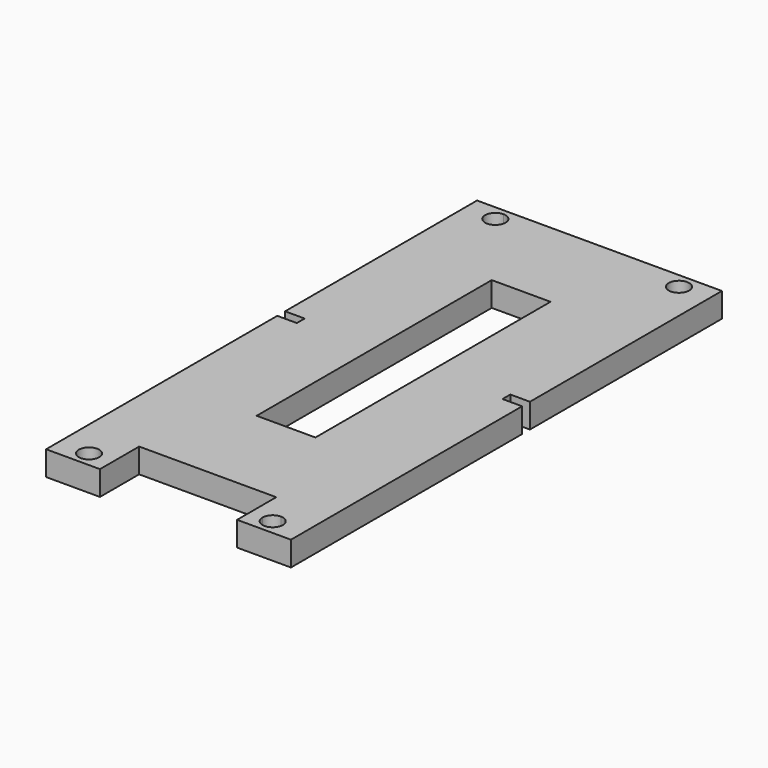
from build123d import *

# Parameters (mm, degrees)
F1_DEPTH  = 3.175
F2_W      = 1.27
F2_H      = 3.175
F3_DEPTH  = 2.54
F4_W      = 1.27
F4_H      = 3.175
F5_DEPTH  = 2.54
F6_W      = 6.985
F6_H      = 3.175
F7_DEPTH  = 6.35
F9_DEPTH  = 25.4
F10_DEPTH = 25.4


# Not quite as in the source:
# - a feature names something its author has since deleted; it is built from what else it names


with BuildPart() as f1:
    # F0 (on Top) → F1 (new body)
    with BuildSketch(Plane.XY):
        Polygon((0, 63.5), (0, 0), (15.875, 0), (15.875, 12.7), (12.065, 12.7), (12.065, 50.8), (15.875, 50.8), (15.875, 63.5), align=None)
        Polygon((15.875, 12.7), (15.875, 0), (31.75, 0), (31.75, 63.5), (15.875, 63.5), (15.875, 50.8), (19.685, 50.8), (19.685, 12.7), align=None)
    extrude(amount=F1_DEPTH)

    # F2 (on face) → F3 (cut)
    with BuildSketch(Plane.YZ.offset(31.75)):
        with Locations((31.75, 1.5875)):
            Rectangle(F2_W, F2_H)
    extrude(amount=-F3_DEPTH, mode=Mode.SUBTRACT)

    # F4 (on face) → F5 (cut)
    with BuildSketch(Plane(origin=(0, 0, 0), x_dir=(0, -1, 0), z_dir=(-1, 0, 0))):
        with Locations((-31.75, 1.5875)):
            Rectangle(F4_W, F4_H)
    extrude(amount=-F5_DEPTH, mode=Mode.SUBTRACT)

    # F6 (on face) → F7 (join)
    with BuildSketch(Plane.XZ):
        with Locations((3.4925, 1.5875)):
            Rectangle(F6_W, F6_H)
        with Locations((28.2575, 1.5875)):
            Rectangle(F6_W, F6_H)
    extrude(amount=F7_DEPTH)

    # F8 (on face) → F9 (cut)
    with BuildSketch(Plane.XY.offset(3.175)):
        with BuildLine():
            ThreePointArc((5.29375, -4.35), (3.0318335149, -3.4130835149), (3.96875, -5.675))
            Line((3.96875, -5.675), (3.96875, -4.35))
            Line((3.96875, -4.35), (5.29375, -4.35))
        make_face()
        with BuildLine():
            Line((3.96875, -4.35), (3.96875, -5.675))
            ThreePointArc((3.96875, -5.675), (4.9056664851, -5.2869164851), (5.29375, -4.35))
            Line((5.29375, -4.35), (3.96875, -4.35))
        make_face()
        with BuildLine():
            ThreePointArc((27.78125, -3.025), (26.8443335149, -3.4130835149), (26.45625, -4.35))
            Line((26.45625, -4.35), (27.78125, -4.35))
            Line((27.78125, -4.35), (27.78125, -3.025))
        make_face()
    extrude(amount=-F9_DEPTH, mode=Mode.SUBTRACT)

    # F8 (on face) → F10 (cut)
    with BuildSketch(Plane.XY.offset(3.175)):
        with BuildLine():
            ThreePointArc((29.10625, 61.5), (27.78125, 62.825), (26.45625, 61.5))
            ThreePointArc((26.45625, 61.5), (27.78125, 60.175), (29.10625, 61.5))
        make_face()
        with BuildLine():
            ThreePointArc((5.29375, 61.5), (4.9056664851, 62.4369164851), (3.96875, 62.825))
            ThreePointArc((3.96875, 62.825), (3.0318335149, 60.5630835149), (5.29375, 61.5))
        make_face()
        with BuildLine():
            Line((27.78125, -4.35), (26.45625, -4.35))
            ThreePointArc((26.45625, -4.35), (26.8443335149, -5.2869164851), (27.78125, -5.675))
            ThreePointArc((27.78125, -5.675), (28.7181664851, -5.2869164851), (29.10625, -4.35))
            ThreePointArc((29.10625, -4.35), (28.7181664851, -3.4130835149), (27.78125, -3.025))
            Line((27.78125, -3.025), (27.78125, -4.35))
        make_face()
    extrude(amount=-F10_DEPTH, mode=Mode.SUBTRACT)


solid = f1.part
